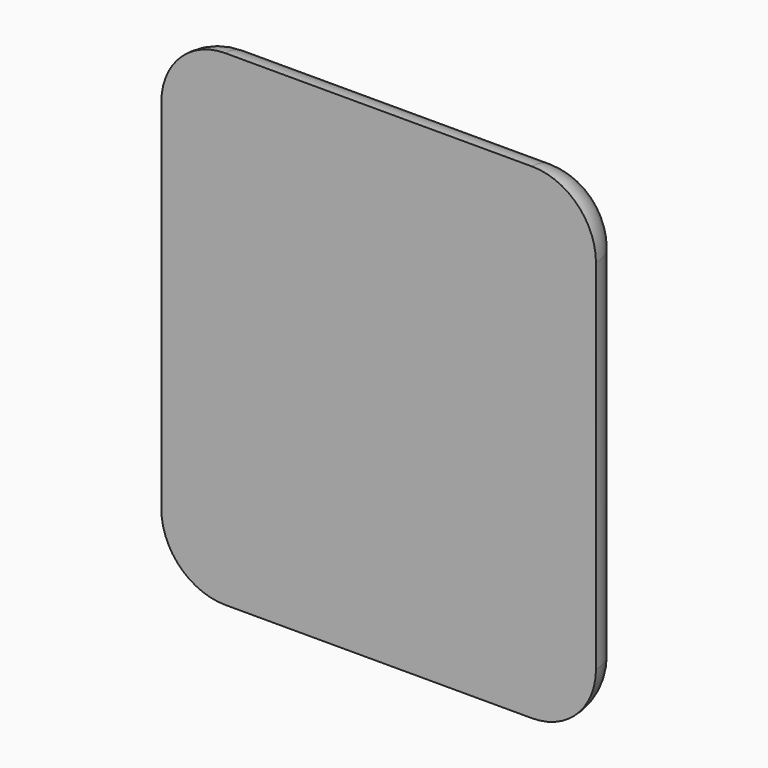
from build123d import *

# Parameters (mm, degrees)
F1_DEPTH = 3
F2_R     = 7.5
F3_DEPTH = 3
F5_DEPTH = 12.5
F6_R     = 2.99999
F7_R     = 1


# Not quite as in the source:
# - a fillet or chamfer is up to 0.001 mm smaller than in the source, because OpenCascade refuses the exact size


with BuildPart() as f1:
    # F0 (on Front) → F1 (new body)
    with BuildSketch(Plane.XZ):
        with BuildLine():
            ThreePointArc((-17, 5), (-15.5355339059, 1.4644660941), (-12, 0))
            Line((-12, 0), (12, 0))
            ThreePointArc((12, 0), (15.5355339059, 1.4644660941), (17, 5))
            Line((17, 5), (17, 33))
            ThreePointArc((17, 33), (15.5355339059, 36.5355339059), (12, 38))
            Line((12, 38), (-12, 38))
            ThreePointArc((-12, 38), (-15.5355339059, 36.5355339059), (-17, 33))
            Line((-17, 33), (-17, 5))
        make_face()
    extrude(amount=F1_DEPTH)

    # F2 (on face) → F3 (join)
    with BuildSketch(Plane(origin=(0, 0, 0), x_dir=(-1, 0, 0), z_dir=(0, 1, 0))):
        with Locations((0, 26)):
            Circle(F2_R)
    extrude(amount=F3_DEPTH)

    # F4 (on Right) → F5 (cut, symmetric)
    with BuildSketch(Plane.YZ):
        Polygon((1.5, 33.5), (0, 33.5), (0, 31.4465926395), (1.504468584, 31.4465926395), align=None)
    extrude(amount=F5_DEPTH, both=True, mode=Mode.SUBTRACT)

    # F6 (radius 3 in the source; OpenCascade refuses exactly that, so slightly less here)
    f6_edges = [f1.edges().sort_by_distance(p)[0] for p in [
        (17, 0, 19),
    ]]
    fillet(f6_edges, radius=F6_R)

    # F7
    f7_edges = [f1.edges().sort_by_distance(p)[0] for p in [
        (7.5, 3, 26),
        (2.964775, 0, 19.11087),
    ]]
    fillet(f7_edges, radius=F7_R)


solid = f1.part
